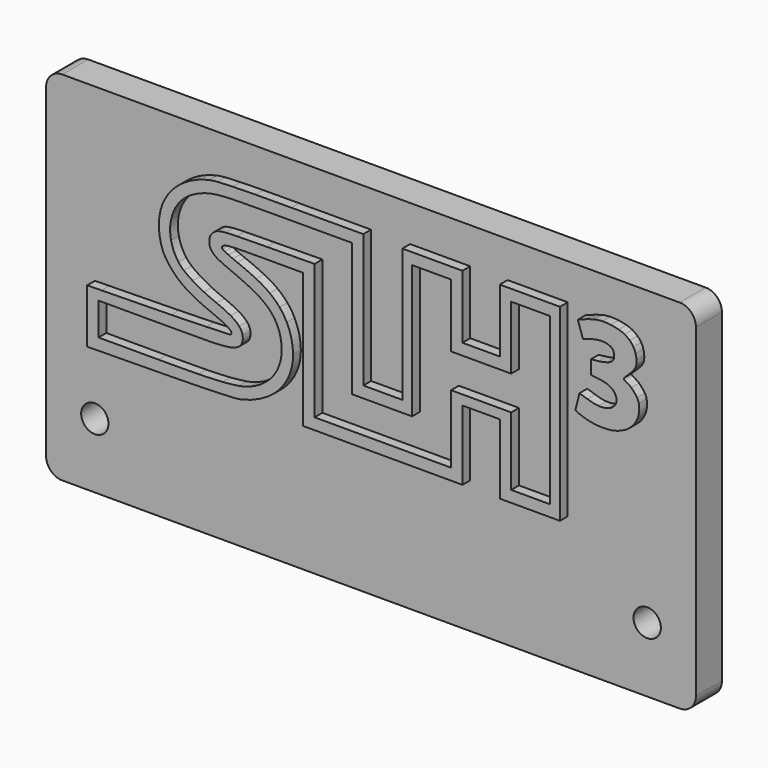
from build123d import *

# Parameters (mm, degrees)
F1_DEPTH = 6
F2_SCALE = 0.25
F3_W     = 100
F3_H     = 55
F3_R     = 2.1
F4_DEPTH = 5
F5_R     = 2.5


# Not quite as in the source:
# - ends of sketch curves that miss each other by under 0.0002 mm in the source are joined


with BuildPart() as f1:
    # F0 (on Front) → F1 (new body)
    with BuildSketch(Plane.XZ):
        with BuildLine():
            ThreePointArc((152.341228018, 58.1349171313), (149.8269064082, 58.3597525344), (147.3038345575, 58.4402047098))
            ThreePointArc((147.3038345575, 58.4402047098), (144.8923426463, 58.2191881424), (142.5041551762, 57.818311393))
            ThreePointArc((142.5041551762, 57.818311393), (141.6286371814, 57.5874283564), (140.7541334629, 57.352732867))
            ThreePointArc((140.7541334629, 57.352732867), (139.7941303297, 57.0530705945), (138.8354301453, 56.749265641))
            ThreePointArc((138.8354301453, 56.749265641), (137.8311964898, 56.4206441356), (136.8284840268, 56.0874099159))
            ThreePointArc((136.8284840268, 56.0874099159), (134.4494339346, 55.2578316154), (132.1058124304, 54.3328896165))
            Line((132.1058124304, 54.3328896165), (135.2964043617, 44.7889044881))
            ThreePointArc((135.2964043617, 44.7889044881), (138.9218950311, 46.1431942866), (142.6777168508, 47.0770496879))
            ThreePointArc((142.6777168508, 47.0770496879), (145.3037154455, 47.4599296937), (147.9574100047, 47.4791820766))
            ThreePointArc((147.9574100047, 47.4791820766), (150.0024260919, 47.1622128392), (151.9545679078, 46.4754067993))
            ThreePointArc((151.9545679078, 46.4754067993), (153.2497169486, 45.5413952884), (154.0946016381, 44.1864198624))
            ThreePointArc((154.0946016381, 44.1864198624), (154.4618796803, 42.6793722604), (154.4471411344, 41.1282859819))
            ThreePointArc((154.4471411344, 41.1282859819), (154.0274505966, 39.8196352665), (153.1810760747, 38.7368809167))
            ThreePointArc((153.1810760747, 38.7368809167), (151.7322273647, 37.7109786626), (150.0881481192, 37.0411715732))
            ThreePointArc((150.0881481192, 37.0411715732), (147.5640252841, 36.4404230958), (145.0010969923, 36.0360800651))
            Line((145.0010969923, 36.0360800651), (140.077451, 35.452947))
            Line((140.077451, 35.452947), (140.077451, 31.231529))
            Line((140.077451, 31.231529), (140.077451, 27.010111))
            Line((140.077451, 27.010111), (145.313272, 26.390005))
            ThreePointArc((145.313272, 26.390005), (147.4995114305, 26.0344391507), (149.6467600868, 25.4909382897))
            ThreePointArc((149.6467600868, 25.4909382897), (151.3253195044, 24.8379266625), (152.8788301944, 23.9265592779))
            ThreePointArc((152.8788301944, 23.9265592779), (154.0260482227, 22.9373393661), (154.9508350367, 21.7375750228))
            ThreePointArc((154.9508350367, 21.7375750228), (155.5731072533, 20.4211762125), (155.8821842516, 18.9982919249))
            ThreePointArc((155.8821842516, 18.9982919249), (155.6792998869, 16.9086609443), (154.6903602154, 15.0567108232))
            ThreePointArc((154.6903602154, 15.0567108232), (152.9583603485, 13.4737955374), (150.8501020813, 12.4438967473))
            ThreePointArc((150.8501020813, 12.4438967473), (147.9002641766, 11.809008744), (144.8831400017, 11.7691580196))
            ThreePointArc((144.8831400017, 11.7691580196), (141.4066010267, 12.2925822347), (138.0238769802, 13.2504309438))
            Line((138.0238769802, 13.2504309438), (133.1239811244, 14.812147956))
            Line((133.1239811244, 14.812147956), (130.5830776691, 4.6951826662))
            ThreePointArc((130.5830776691, 4.6951826662), (134.3545111151, 3.0830213335), (138.2702710743, 1.8625303084))
            ThreePointArc((138.2702710743, 1.8625303084), (144.6475148349, 0.8652287383), (151.1020819971, 0.9143360329))
            ThreePointArc((151.1020819971, 0.9143360329), (156.7168065495, 2.0783580357), (161.91616203, 4.4963699511))
            ThreePointArc((161.91616203, 4.4963699511), (165.7064525048, 7.6555621469), (168.4426272472, 11.7616728825))
            ThreePointArc((168.4426272472, 11.7616728825), (169.7953031287, 16.3544948874), (169.6605109651, 21.1404719934))
            ThreePointArc((169.6605109651, 21.1404719934), (169.2435398041, 22.6044121534), (168.5656666596, 23.9673037896))
            ThreePointArc((168.5656666596, 23.9673037896), (166.9064128382, 26.1972938101), (165.0162637234, 28.2352622598))
            ThreePointArc((165.0162637234, 28.2352622598), (162.9669138924, 29.6544963373), (160.7904410002, 30.8698258589))
            ThreePointArc((160.7904410002, 30.8698258589), (160.3825279534, 31.451864804), (160.663634351, 32.1046600097))
            ThreePointArc((160.663634351, 32.1046600097), (162.3630635173, 33.8079757087), (164.0774507347, 35.4962352653))
            ThreePointArc((164.0774507347, 35.4962352653), (165.1707236148, 36.6322034695), (166.2196933125, 37.809204732))
            ThreePointArc((166.2196933125, 37.809204732), (166.8414404287, 38.6357965203), (167.3527699769, 39.5348880112))
            ThreePointArc((167.3527699769, 39.5348880112), (167.8080801222, 40.4998853929), (168.087775057, 41.5295931274))
            ThreePointArc((168.087775057, 41.5295931274), (168.1977643706, 42.8800995541), (168.1963354349, 44.2350767553))
            ThreePointArc((168.1963354349, 44.2350767553), (167.9958020572, 45.8752345594), (167.6282000052, 47.4861970012))
            ThreePointArc((167.6282000052, 47.4861970012), (167.0891813187, 49.1526573167), (166.3039485131, 50.7182373082))
            ThreePointArc((166.3039485131, 50.7182373082), (165.2790917625, 52.1671747641), (164.0500026364, 53.4474447096))
            ThreePointArc((164.0500026364, 53.4474447096), (162.513830675, 54.6803953844), (160.8520869325, 55.7380338798))
            ThreePointArc((160.8520869325, 55.7380338798), (159.1271747087, 56.5645242409), (157.3094311562, 57.1596856085))
            ThreePointArc((157.3094311562, 57.1596856085), (154.8393231071, 57.7185897611), (152.341228018, 58.1349171313))
        make_face()
    extrude(amount=F1_DEPTH)


with BuildPart() as f1b:
    # F0 (on Front) → F1, piece 2 (new body)
    with BuildSketch(Plane.XZ):
        with BuildLine():
            ThreePointArc((-89.7158710092, 56.8834551585), (-92.2735942046, 56.6347400971), (-94.8042470377, 56.1879701736))
            ThreePointArc((-94.8042470377, 56.1879701736), (-99.3736938541, 54.9568862269), (-103.7987699924, 53.2793543903))
            ThreePointArc((-103.7987699924, 53.2793543903), (-107.8572904997, 51.2349120693), (-111.665558992, 48.7553104477))
            ThreePointArc((-111.665558992, 48.7553104477), (-115.0425226555, 45.9681171918), (-118.0767520571, 42.8112545453))
            ThreePointArc((-118.0767520571, 42.8112545453), (-121.12070834, 38.6532182392), (-123.4993151686, 34.0818764963))
            ThreePointArc((-123.4993151686, 34.0818764963), (-125.7717067995, 20.9710825795), (-123.0967220919, 7.9364695178))
            ThreePointArc((-123.0967220919, 7.9364695178), (-120.9885218169, 4.3857057485), (-118.5278910102, 1.0694235263))
            ThreePointArc((-118.5278910102, 1.0694235263), (-115.7462308189, -1.9692311529), (-112.6660909179, -4.7048835193))
            ThreePointArc((-112.6660909179, -4.7048835193), (-108.9951941367, -7.3754936141), (-105.0961528177, -9.7003846329))
            ThreePointArc((-105.0961528177, -9.7003846329), (-100.2941341921, -12.1054997132), (-95.3662908353, -14.2409905891))
            ThreePointArc((-95.3662908353, -14.2409905891), (-91.8421068748, -15.6870234447), (-88.3419598235, -17.1903045981))
            ThreePointArc((-88.3419598235, -17.1903045981), (-86.1529724976, -18.2297863885), (-84.0291443228, -19.3966375486))
            ThreePointArc((-84.0291443228, -19.3966375486), (-82.7599951917, -20.2264826141), (-81.5746631598, -21.172194182))
            ThreePointArc((-81.5746631598, -21.172194182), (-81.1710412365, -21.8195919106), (-81.1923597658, -22.5822060778))
            ThreePointArc((-81.1923597658, -22.5822060778), (-81.6047236673, -23.1553562233), (-82.2701210101, -23.3915577353))
            ThreePointArc((-82.2701210101, -23.3915577353), (-89.4196222871, -23.6529407729), (-96.5698990129, -23.8921735944))
            ThreePointArc((-96.5698990129, -23.8921735944), (-107.3762638319, -24.1981884626), (-118.1845449963, -24.426714213))
            ThreePointArc((-118.1845449963, -24.426714213), (-139.6783524604, -24.7922369482), (-161.1725489962, -25.1341162467))
            Line((-161.1725489962, -25.1341162467), (-169.922549, -25.268471))
            Line((-169.922549, -25.268471), (-169.922549, -41.902849))
            Line((-169.922549, -41.902849), (-169.922549, -58.537228))
            Line((-169.922549, -58.537228), (-125.172549, -58.013692))
            ThreePointArc((-125.172549, -58.013692), (-115.0424725161, -57.8782248746), (-104.9129060058, -57.7088636826))
            ThreePointArc((-104.9129060058, -57.7088636826), (-97.5129944762, -57.5418252197), (-90.114737023, -57.3129603439))
            ThreePointArc((-90.114737023, -57.3129603439), (-84.6913364364, -57.1009616803), (-79.2697880179, -56.8459516498))
            ThreePointArc((-79.2697880179, -56.8459516498), (-77.083403988, -56.6404610548), (-74.9225491136, -56.2490434966))
            ThreePointArc((-74.9225491136, -56.2490434966), (-66.2429199717, -53.4275060959), (-58.229199749, -49.0597463737))
            ThreePointArc((-58.229199749, -49.0597463737), (-51.8949561555, -43.6034600395), (-47.0349944418, -36.8009257582))
            ThreePointArc((-47.0349944418, -36.8009257582), (-44.1187465301, -29.3501508182), (-43.1776257233, -21.4045329973))
            ThreePointArc((-43.1776257233, -21.4045329973), (-44.2002643647, -13.1406454463), (-47.0554066795, -5.3185108399))
            ThreePointArc((-47.0554066795, -5.3185108399), (-49.0771830946, -1.8182961093), (-51.5059305748, 1.4128443618))
            ThreePointArc((-51.5059305748, 1.4128443618), (-54.3478662536, 4.3900005354), (-57.5111356244, 7.0232085076))
            ThreePointArc((-57.5111356244, 7.0232085076), (-61.5514455995, 9.7367639846), (-65.8219646825, 12.0713206495))
            ThreePointArc((-65.8219646825, 12.0713206495), (-71.5688253864, 14.7325295165), (-77.4225488118, 17.1496274843))
            ThreePointArc((-77.4225488118, 17.1496274843), (-78.8401462889, 17.7131254267), (-80.2487799398, 18.2986711417))
            ThreePointArc((-80.2487799398, 18.2986711417), (-81.6057167765, 18.888922599), (-82.9523677552, 19.5022785255))
            ThreePointArc((-82.9523677552, 19.5022785255), (-84.0942604495, 20.0454792956), (-85.2272229395, 20.6070681197))
            ThreePointArc((-85.2272229395, 20.6070681197), (-85.8377507575, 20.9485781165), (-86.4176780147, 21.3398039801))
            ThreePointArc((-86.4176780147, 21.3398039801), (-86.853730235, 22.0915551847), (-86.6016505259, 22.9232565972))
            ThreePointArc((-86.6016505259, 22.9232565972), (-85.6588933579, 23.6905603449), (-84.5036700444, 24.0687213317))
            ThreePointArc((-84.5036700444, 24.0687213317), (-80.9344247322, 24.4386370453), (-77.3495189905, 24.5961183335))
            ThreePointArc((-77.3495189905, 24.5961183335), (-69.2612379194, 24.6836352737), (-61.1725489995, 24.7162152783))
            Line((-61.1725489995, 24.7162152783), (-36.922549, 24.731529))
            Line((-36.922549, 24.731529), (-36.922549, -16.768471))
            Line((-36.922549, -16.768471), (-36.922549, -58.268471))
            Line((-36.922549, -58.268471), (12.077451, -58.268471))
            Line((12.077451, -58.268471), (61.077451, -58.268471))
            Line((61.077451, -58.268471), (61.077451, -36.768471))
            Line((61.077451, -36.768471), (61.077451, -15.268471))
            Line((61.077451, -15.268471), (72.577451, -15.268471))
            Line((72.577451, -15.268471), (84.077451, -15.268471))
            Line((84.077451, -15.268471), (84.077451, -36.768471))
            Line((84.077451, -36.768471), (84.077451, -58.268471))
            Line((84.077451, -58.268471), (102.577451, -58.268471))
            Line((102.577451, -58.268471), (121.077451, -58.268471))
            Line((121.077451, -58.268471), (121.077451, -0.268471))
            Line((121.077451, -0.268471), (121.077451, 57.731529))
            Line((121.077451, 57.731529), (102.577451, 57.731529))
            Line((102.577451, 57.731529), (84.077451, 57.731529))
            Line((84.077451, 57.731529), (84.077451, 38.231529))
            Line((84.077451, 38.231529), (84.077451, 18.731529))
            Line((84.077451, 18.731529), (72.577451, 18.731529))
            Line((72.577451, 18.731529), (61.077451, 18.731529))
            Line((61.077451, 18.731529), (61.077451, 38.231529))
            Line((61.077451, 38.231529), (61.077451, 57.731529))
            Line((61.077451, 57.731529), (42.577451, 57.731529))
            Line((42.577451, 57.731529), (24.077451, 57.731529))
            Line((24.077451, 57.731529), (24.077451, 16.731529))
            Line((24.077451, 16.731529), (24.077451, -24.268471))
            Line((24.077451, -24.268471), (12.077451, -24.268471))
            Line((12.077451, -24.268471), (0.077451, -24.268471))
            Line((0.077451, -24.268471), (0.077451, 16.731529))
            Line((0.077451, 16.731529), (0.077451, 57.731529))
            Line((0.077451, 57.731529), (-44.172549, 57.652029))
            ThreePointArc((-44.172549, 57.652029), (-55.2418806461, 57.6161162906), (-66.3110620044, 57.5481685759))
            ThreePointArc((-66.3110620044, 57.5481685759), (-73.3088995976, 57.4577720999), (-80.3053760072, 57.2927862479))
            ThreePointArc((-80.3053760072, 57.2927862479), (-85.0121136593, 57.1223791714), (-89.7158710092, 56.8834551585))
        make_face()
        with BuildLine():
            Line((-6.922549, 50.731529), (-6.922549, 9.731529))
            Line((-6.922549, 9.731529), (-6.922549, -31.268471))
            Line((-6.922549, -31.268471), (11.577451, -31.268471))
            Line((11.577451, -31.268471), (30.077451, -31.268471))
            Line((30.077451, -31.268471), (30.077451, 9.731529))
            Line((30.077451, 9.731529), (30.077451, 50.731529))
            Line((30.077451, 50.731529), (42.077451, 50.731529))
            Line((42.077451, 50.731529), (54.077451, 50.731529))
            Line((54.077451, 50.731529), (54.077451, 31.231529))
            Line((54.077451, 31.231529), (54.077451, 11.731529))
            Line((54.077451, 11.731529), (72.577451, 11.731529))
            Line((72.577451, 11.731529), (91.077451, 11.731529))
            Line((91.077451, 11.731529), (91.077451, 31.231529))
            Line((91.077451, 31.231529), (91.077451, 50.731529))
            Line((91.077451, 50.731529), (103.077451, 50.731529))
            Line((103.077451, 50.731529), (115.077451, 50.731529))
            Line((115.077451, 50.731529), (115.077451, -0.268471))
            Line((115.077451, -0.268471), (115.077451, -51.268471))
            Line((115.077451, -51.268471), (103.077451, -51.268471))
            Line((103.077451, -51.268471), (91.077451, -51.268471))
            Line((91.077451, -51.268471), (91.077451, -30.268471))
            Line((91.077451, -30.268471), (91.077451, -9.268471))
            Line((91.077451, -9.268471), (72.577451, -9.268471))
            Line((72.577451, -9.268471), (54.077451, -9.268471))
            Line((54.077451, -9.268471), (54.077451, -30.268471))
            Line((54.077451, -30.268471), (54.077451, -51.268471))
            Line((54.077451, -51.268471), (12.077451, -51.268471))
            Line((12.077451, -51.268471), (-29.922549, -51.268471))
            Line((-29.922549, -51.268471), (-29.922549, -9.712924))
            Line((-29.922549, -9.712924), (-29.922549, 31.842624))
            Line((-29.922549, 31.842624), (-59.351393, 31.537076))
            ThreePointArc((-59.351393, 31.537076), (-68.5850462649, 31.4296314933), (-77.8184010104, 31.2990286783))
            ThreePointArc((-77.8184010104, 31.2990286783), (-81.409671871, 31.1906978742), (-84.9961810646, 30.9764228658))
            ThreePointArc((-84.9961810646, 30.9764228658), (-86.9969034513, 30.7468714781), (-88.9730370675, 30.3589542835))
            ThreePointArc((-88.9730370675, 30.3589542835), (-90.3497041231, 29.8794538341), (-91.6013931015, 29.1321871364))
            ThreePointArc((-91.6013931015, 29.1321871364), (-92.2881410377, 28.5718283118), (-92.9221711737, 27.9524491626))
            ThreePointArc((-92.9221711737, 27.9524491626), (-93.4234380719, 27.3440152924), (-93.8438617689, 26.677153874))
            ThreePointArc((-93.8438617689, 26.677153874), (-94.1817162815, 25.9538613819), (-94.4271884372, 25.1942291118))
            ThreePointArc((-94.4271884372, 25.1942291118), (-94.6171600755, 24.2984091052), (-94.7324511912, 23.3899540163))
            ThreePointArc((-94.7324511912, 23.3899540163), (-94.6898825108, 21.7428303685), (-94.2866406888, 20.1452621164))
            ThreePointArc((-94.2866406888, 20.1452621164), (-93.5430426827, 18.6793780125), (-92.4936754461, 17.414236537))
            ThreePointArc((-92.4936754461, 17.414236537), (-90.8288592178, 16.0278457455), (-88.9812839954, 14.8964050088))
            ThreePointArc((-88.9812839954, 14.8964050088), (-86.0853857569, 13.4838421599), (-83.127087951, 12.2071141212))
            ThreePointArc((-83.127087951, 12.2071141212), (-76.1046774408, 9.2216982414), (-69.192652154, 5.9889186855))
            ThreePointArc((-69.192652154, 5.9889186855), (-64.6346128235, 3.4496167949), (-60.3711449209, 0.4418571004))
            ThreePointArc((-60.3711449209, 0.4418571004), (-57.3596650438, -2.3287384368), (-54.8044534441, -5.5250026212))
            ThreePointArc((-54.8044534441, -5.5250026212), (-52.7953245926, -9.0398392377), (-51.3626788706, -12.8264209624))
            ThreePointArc((-51.3626788706, -12.8264209624), (-50.3291791157, -18.119537933), (-50.2608906295, -23.5121759512))
            ThreePointArc((-50.2608906295, -23.5121759512), (-51.1807718794, -28.6284665045), (-53.1033518636, -33.4581970709))
            ThreePointArc((-53.1033518636, -33.4581970709), (-55.9945311141, -37.8976652666), (-59.6944190526, -41.6895809375))
            ThreePointArc((-59.6944190526, -41.6895809375), (-64.2892009878, -44.9586351909), (-69.3529080105, -47.4400879732))
            ThreePointArc((-69.3529080105, -47.4400879732), (-72.8684407738, -48.6039602475), (-76.4898430612, -49.3779206108))
            ThreePointArc((-76.4898430612, -49.3779206108), (-81.4935417039, -50.0516975389), (-86.5221440209, -50.5035096908))
            ThreePointArc((-86.5221440209, -50.5035096908), (-93.9698805478, -50.9055572117), (-101.4257790076, -51.1055564262))
            ThreePointArc((-101.4257790076, -51.1055564262), (-113.71007347, -51.2277373319), (-125.994908, -51.2684709995))
            Line((-125.994908, -51.2684709995), (-162.922549, -51.268471))
            Line((-162.922549, -51.268471), (-162.922549, -41.268471))
            Line((-162.922549, -41.268471), (-162.922549, -31.268471))
            Line((-162.922549, -31.268471), (-122.89043, -31.268471))
            ThreePointArc((-122.89043, -31.268471), (-108.6116969212, -31.2385282409), (-94.333215, -31.148701002))
            ThreePointArc((-94.333215, -31.148701002), (-88.8830809379, -30.9627118289), (-83.4497240276, -30.4966797533))
            ThreePointArc((-83.4497240276, -30.4966797533), (-80.5892836984, -29.9451631776), (-77.8516171162, -28.9494367453))
            ThreePointArc((-77.8516171162, -28.9494367453), (-76.0486360653, -27.6977755498), (-74.7978693807, -25.8941738265))
            ThreePointArc((-74.7978693807, -25.8941738265), (-74.163782837, -23.6465963892), (-74.2341387938, -21.3123469619))
            ThreePointArc((-74.2341387938, -21.3123469619), (-74.9963742674, -19.0247201541), (-76.3569290939, -17.0339590855))
            ThreePointArc((-76.3569290939, -17.0339590855), (-78.7940710577, -14.772962488), (-81.5764459433, -12.9535788949))
            ThreePointArc((-81.5764459433, -12.9535788949), (-85.8570506833, -10.8047203157), (-90.2567551169, -8.9116352955))
            ThreePointArc((-90.2567551169, -8.9116352955), (-94.2221619869, -7.2543553332), (-98.1217563571, -5.4476477338))
            ThreePointArc((-98.1217563571, -5.4476477338), (-101.5861180366, -3.6519049869), (-104.9550017172, -1.6828655431))
            ThreePointArc((-104.9550017172, -1.6828655431), (-107.7122197443, 0.1346344078), (-110.3613500245, 2.106350969))
            ThreePointArc((-110.3613500245, 2.106350969), (-112.1670046714, 3.7461922987), (-113.7300718859, 5.6187010826))
            ThreePointArc((-113.7300718859, 5.6187010826), (-116.5390282465, 10.4950047459), (-118.280515566, 15.8462470928))
            ThreePointArc((-118.280515566, 15.8462470928), (-118.8790101532, 21.4407000717), (-118.3086948317, 27.0380959649))
            ThreePointArc((-118.3086948317, 27.0380959649), (-116.5989502708, 32.3696733886), (-113.8179953448, 37.2292242485))
            ThreePointArc((-113.8179953448, 37.2292242485), (-110.1022751062, 41.3715968897), (-105.5938670631, 44.6335111102))
            ThreePointArc((-105.5938670631, 44.6335111102), (-101.8608058475, 46.5327187651), (-97.9596561103, 48.0571093289))
            ThreePointArc((-97.9596561103, 48.0571093289), (-94.0658785153, 49.1295336068), (-90.0782940356, 49.7704453392))
            ThreePointArc((-90.0782940356, 49.7704453392), (-83.9399176718, 50.2700740279), (-77.7848659949, 50.4813365343))
            ThreePointArc((-77.7848659949, 50.4813365343), (-62.9789210123, 50.6078184187), (-48.1725489998, 50.6657178536))
            Line((-48.1725489998, 50.6657178536), (-6.922549, 50.731529))
        make_face(mode=Mode.SUBTRACT)
    extrude(amount=F1_DEPTH)


with BuildPart() as f1_1:
    # F2: moved
    add(f1.part.scale(F2_SCALE))


with BuildPart() as f1b_1:
    # F2: moved
    add(f1b.part.scale(F2_SCALE))


with BuildPart() as f4:
    # F3 (on Front) → F4 (new body)
    with BuildSketch(Plane.XZ):
        with Locations((0, -7.5)):
            Rectangle(F3_W, F3_H)
        with Locations((-42.5, -25)):
            Circle(F3_R, mode=Mode.SUBTRACT)
        with Locations((42.5, -25)):
            Circle(F3_R, mode=Mode.SUBTRACT)
    extrude(amount=-F4_DEPTH)

    # F5
    f5_edges = [f4.edges().sort_by_distance(p)[0] for p in [
        (-50, 2.5, 20),
        (-50, 2.5, -35),
        (50, 2.5, -35),
        (50, 2.5, 20),
    ]]
    fillet(f5_edges, radius=F5_R)


solid = Compound([f1_1.part, f1b_1.part, f4.part])
